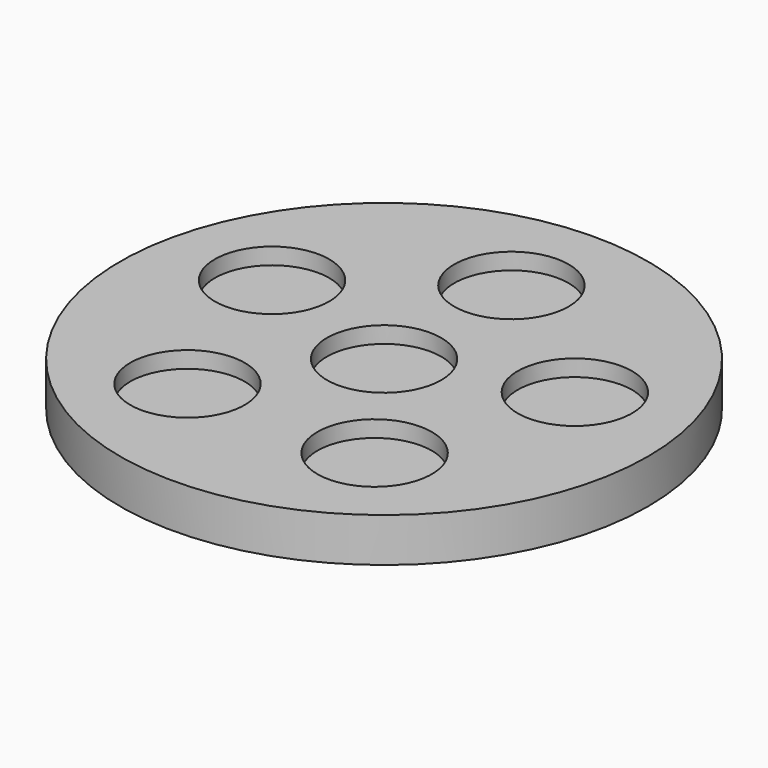
from build123d import *

# Parameters (mm, degrees)
F0_R            = 76.2
F1_DEPTH        = 12.7
F2_R            = 16.51
F3_DEPTH        = 4.7625
F3_COPIES_COUNT = 5
F4_R            = 16.51
F5_DEPTH        = 4.7625


# Not quite as in the source:
# - a pattern or mirror of a feature is missing from the dataset's text; its kind, count and spacing are read off the source's solid


with BuildPart() as f1:
    # F0 (on Top) → F1 (new body)
    with BuildSketch(Plane.XY):
        Circle(F0_R)
    extrude(amount=F1_DEPTH)

    # F2 (on face) → F3 (cut)
    with BuildSketch(Plane.XY.offset(12.7)):
        with Locations((0, 45.9601860202)):
            Circle(F2_R)
    f3 = extrude(amount=-F3_DEPTH, mode=Mode.SUBTRACT)

    # F3_copies: F3 ×5 about axis
    f3_copies_axis = Axis((0, 0, 0), (0, 0, 1))
    for i in range(1, F3_COPIES_COUNT):
        add(f3.rotate(f3_copies_axis, i * 360 / F3_COPIES_COUNT), mode=Mode.SUBTRACT)

    # F4 (on face) → F5 (cut)
    with BuildSketch(Plane.XY.offset(12.7)):
        Circle(F4_R)
    extrude(amount=-F5_DEPTH, mode=Mode.SUBTRACT)


solid = f1.part
